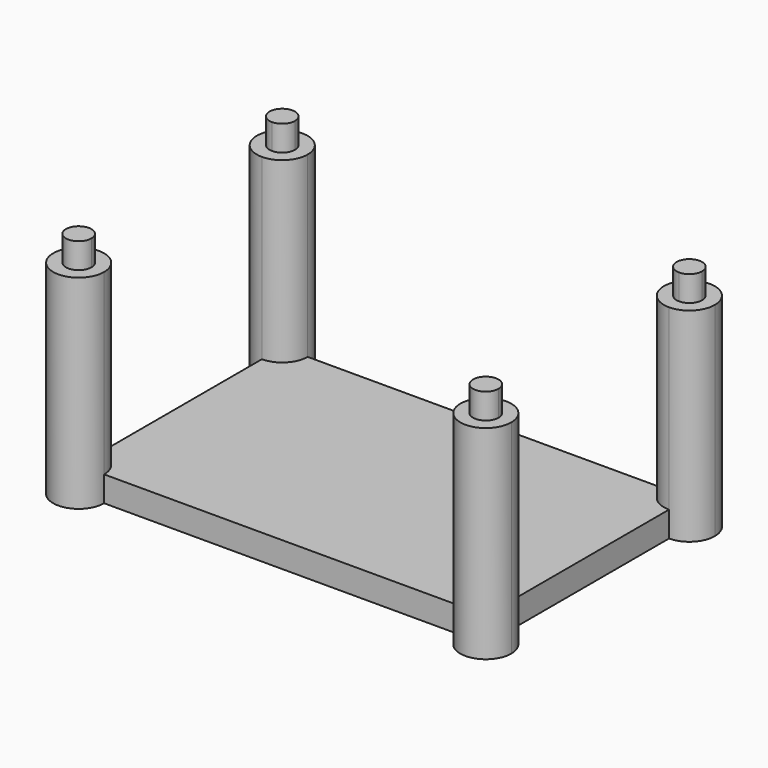
from build123d import *

# Parameters (mm, degrees)
F1_DEPTH   = 50.8
F2_DEPTH   = 6.35
F3_DEPTH   = 57.15
F4_D       = 7.62
F4_DEPTH   = 7.62
F4_TIP     = 2.2892789585
F4_2_D     = 7.62
F4_2_DEPTH = 7.62
F4_2_TIP   = 2.2892789585
F4_3_D     = 7.62
F4_3_DEPTH = 7.62
F4_3_TIP   = 2.2892789585
F4_4_D     = 7.62
F4_4_DEPTH = 7.62
F4_4_TIP   = 2.2892789585
F4_5_D     = 7.62
F4_5_DEPTH = 7.62
F4_5_TIP   = 2.2892789585
F4_6_D     = 7.62
F4_6_DEPTH = 7.62
F4_6_TIP   = 2.2892789585
F4_7_D     = 7.62
F4_7_DEPTH = 7.62
F4_7_TIP   = 2.2892789585
F4_8_D     = 7.62
F4_8_DEPTH = 7.62
F4_8_TIP   = 2.2892789585


with BuildPart() as f1:
    # F0 (on Top) → F1 (new body)
    with BuildSketch(Plane.XY):
        with BuildLine():
            Line((-47.625, 31.75), (-44.45, 31.75))
            ThreePointArc((-44.45, 31.75), (-55.2901280605, 36.2401280605), (-50.8, 25.4))
            Line((-50.8, 25.4), (-50.8, 28.575))
            ThreePointArc((-50.8, 28.575), (-53.0450640303, 33.9950640303), (-47.625, 31.75))
        make_face()
        with BuildLine():
            Line((-50.8, 31.75), (-47.625, 31.75))
            ThreePointArc((-47.625, 31.75), (-53.0450640303, 33.9950640303), (-50.8, 28.575))
            Line((-50.8, 28.575), (-50.8, 31.75))
        make_face()
        with BuildLine():
            ThreePointArc((-50.8, 28.575), (-48.5549359697, 29.5049359697), (-47.625, 31.75))
            Line((-47.625, 31.75), (-50.8, 31.75))
            Line((-50.8, 31.75), (-50.8, 28.575))
        make_face()
        with BuildLine():
            ThreePointArc((-50.8, 25.4), (-46.3098719395, 27.2598719395), (-44.45, 31.75))
            Line((-44.45, 31.75), (-47.625, 31.75))
            ThreePointArc((-47.625, 31.75), (-48.5549359697, 29.5049359697), (-50.8, 28.575))
            Line((-50.8, 28.575), (-50.8, 25.4))
        make_face()
    extrude(amount=F1_DEPTH)

    # F4
    with Locations(Plane(origin=(0, 0, 0), x_dir=(1, 0, 0), z_dir=(0, 0, -1))):
        with Locations((-50.8, 31.75), (-50.8, -31.75), (50.8, -31.75), (50.8, 31.75)):
            Hole(F4_D / 2, depth=F4_DEPTH)
            with Locations((0, 0, -(F4_DEPTH + F4_TIP / 2))):  # 118° drill point
                Cone(0, F4_D / 2, F4_TIP, mode=Mode.SUBTRACT)


with BuildPart() as f1b:
    # F0 (on Top) → F1, piece 2 (new body)
    with BuildSketch(Plane.XY):
        with BuildLine():
            Line((47.625, 31.75), (44.45, 31.75))
            ThreePointArc((44.45, 31.75), (46.3098719395, 27.2598719395), (50.8, 25.4))
            Line((50.8, 25.4), (50.8, 28.575))
            ThreePointArc((50.8, 28.575), (48.5549359697, 29.5049359697), (47.625, 31.75))
        make_face()
        with BuildLine():
            Line((50.8, 31.75), (47.625, 31.75))
            ThreePointArc((47.625, 31.75), (48.5549359697, 29.5049359697), (50.8, 28.575))
            Line((50.8, 28.575), (50.8, 31.75))
        make_face()
        with BuildLine():
            ThreePointArc((57.15, 31.75), (50.8, 38.1), (44.45, 31.75))
            Line((44.45, 31.75), (47.625, 31.75))
            ThreePointArc((47.625, 31.75), (50.8, 34.925), (53.975, 31.75))
            ThreePointArc((53.975, 31.75), (53.0450640303, 29.5049359697), (50.8, 28.575))
            Line((50.8, 28.575), (50.8, 25.4))
            ThreePointArc((50.8, 25.4), (55.2901280605, 27.2598719395), (57.15, 31.75))
        make_face()
        with BuildLine():
            ThreePointArc((53.975, 31.75), (50.8, 34.925), (47.625, 31.75))
            Line((47.625, 31.75), (50.8, 31.75))
            Line((50.8, 31.75), (50.8, 28.575))
            ThreePointArc((50.8, 28.575), (53.0450640303, 29.5049359697), (53.975, 31.75))
        make_face()
    extrude(amount=F1_DEPTH)

    # F4#2
    with Locations(Plane(origin=(0, 0, 0), x_dir=(1, 0, 0), z_dir=(0, 0, -1))):
        with Locations((-50.8, 31.75), (-50.8, -31.75), (50.8, -31.75), (50.8, 31.75)):
            Hole(F4_2_D / 2, depth=F4_2_DEPTH)
            with Locations((0, 0, -(F4_2_DEPTH + F4_2_TIP / 2))):  # 118° drill point
                Cone(0, F4_2_D / 2, F4_2_TIP, mode=Mode.SUBTRACT)


with BuildPart() as f1c:
    # F0 (on Top) → F1, piece 3 (new body)
    with BuildSketch(Plane.XY):
        with BuildLine():
            Line((50.8, -28.575), (50.8, -25.4))
            ThreePointArc((50.8, -25.4), (46.3098719395, -27.2598719395), (44.45, -31.75))
            Line((44.45, -31.75), (47.625, -31.75))
            ThreePointArc((47.625, -31.75), (48.5549359697, -29.5049359697), (50.8, -28.575))
        make_face()
        with BuildLine():
            ThreePointArc((57.15, -31.75), (55.2901280605, -27.2598719395), (50.8, -25.4))
            Line((50.8, -25.4), (50.8, -28.575))
            ThreePointArc((50.8, -28.575), (53.0450640303, -29.5049359697), (53.975, -31.75))
            ThreePointArc((53.975, -31.75), (50.8, -34.925), (47.625, -31.75))
            Line((47.625, -31.75), (44.45, -31.75))
            ThreePointArc((44.45, -31.75), (50.8, -38.1), (57.15, -31.75))
        make_face()
        with BuildLine():
            ThreePointArc((53.975, -31.75), (53.0450640303, -29.5049359697), (50.8, -28.575))
            Line((50.8, -28.575), (50.8, -31.75))
            Line((50.8, -31.75), (47.625, -31.75))
            ThreePointArc((47.625, -31.75), (50.8, -34.925), (53.975, -31.75))
        make_face()
        with BuildLine():
            Line((50.8, -31.75), (50.8, -28.575))
            ThreePointArc((50.8, -28.575), (48.5549359697, -29.5049359697), (47.625, -31.75))
            Line((47.625, -31.75), (50.8, -31.75))
        make_face()
    extrude(amount=F1_DEPTH)

    # F4#3
    with Locations(Plane(origin=(0, 0, 0), x_dir=(1, 0, 0), z_dir=(0, 0, -1))):
        with Locations((-50.8, 31.75), (-50.8, -31.75), (50.8, -31.75), (50.8, 31.75)):
            Hole(F4_3_D / 2, depth=F4_3_DEPTH)
            with Locations((0, 0, -(F4_3_DEPTH + F4_3_TIP / 2))):  # 118° drill point
                Cone(0, F4_3_D / 2, F4_3_TIP, mode=Mode.SUBTRACT)


with BuildPart() as f1d:
    # F0 (on Top) → F1, piece 4 (new body)
    with BuildSketch(Plane.XY):
        with BuildLine():
            Line((-50.8, -28.575), (-50.8, -25.4))
            ThreePointArc((-50.8, -25.4), (-55.2901280605, -36.2401280605), (-44.45, -31.75))
            Line((-44.45, -31.75), (-47.625, -31.75))
            ThreePointArc((-47.625, -31.75), (-53.0450640303, -33.9950640303), (-50.8, -28.575))
        make_face()
        with BuildLine():
            Line((-50.8, -31.75), (-50.8, -28.575))
            ThreePointArc((-50.8, -28.575), (-53.0450640303, -33.9950640303), (-47.625, -31.75))
            Line((-47.625, -31.75), (-50.8, -31.75))
        make_face()
        with BuildLine():
            ThreePointArc((-47.625, -31.75), (-48.5549359697, -29.5049359697), (-50.8, -28.575))
            Line((-50.8, -28.575), (-50.8, -31.75))
            Line((-50.8, -31.75), (-47.625, -31.75))
        make_face()
        with BuildLine():
            ThreePointArc((-44.45, -31.75), (-46.3098719395, -27.2598719395), (-50.8, -25.4))
            Line((-50.8, -25.4), (-50.8, -28.575))
            ThreePointArc((-50.8, -28.575), (-48.5549359697, -29.5049359697), (-47.625, -31.75))
            Line((-47.625, -31.75), (-44.45, -31.75))
        make_face()
    extrude(amount=F1_DEPTH)

    # F4#4
    with Locations(Plane(origin=(0, 0, 0), x_dir=(1, 0, 0), z_dir=(0, 0, -1))):
        with Locations((-50.8, 31.75), (-50.8, -31.75), (50.8, -31.75), (50.8, 31.75)):
            Hole(F4_4_D / 2, depth=F4_4_DEPTH)
            with Locations((0, 0, -(F4_4_DEPTH + F4_4_TIP / 2))):  # 118° drill point
                Cone(0, F4_4_D / 2, F4_4_TIP, mode=Mode.SUBTRACT)


with BuildPart() as f2:
    # F0 (on Top) → F2 (new body)
    with BuildSketch(Plane.XY):
        with BuildLine():
            Line((44.45, 31.75), (-44.45, 31.75))
            ThreePointArc((-44.45, 31.75), (-46.3098719395, 27.2598719395), (-50.8, 25.4))
            Line((-50.8, 25.4), (-50.8, -25.4))
            ThreePointArc((-50.8, -25.4), (-46.3098719395, -27.2598719395), (-44.45, -31.75))
            Line((-44.45, -31.75), (44.45, -31.75))
            ThreePointArc((44.45, -31.75), (46.3098719395, -27.2598719395), (50.8, -25.4))
            Line((50.8, -25.4), (50.8, 25.4))
            ThreePointArc((50.8, 25.4), (46.3098719395, 27.2598719395), (44.45, 31.75))
        make_face()
    extrude(amount=F2_DEPTH)


with BuildPart() as f3:
    # F0 (on Top) → F3 (new body)
    with BuildSketch(Plane.XY):
        with BuildLine():
            Line((-50.8, -31.75), (-50.8, -28.575))
            ThreePointArc((-50.8, -28.575), (-53.0450640303, -33.9950640303), (-47.625, -31.75))
            Line((-47.625, -31.75), (-50.8, -31.75))
        make_face()
        with BuildLine():
            ThreePointArc((-47.625, -31.75), (-48.5549359697, -29.5049359697), (-50.8, -28.575))
            Line((-50.8, -28.575), (-50.8, -31.75))
            Line((-50.8, -31.75), (-47.625, -31.75))
        make_face()
    extrude(amount=F3_DEPTH)

    # F4#5
    with Locations(Plane(origin=(0, 0, 0), x_dir=(1, 0, 0), z_dir=(0, 0, -1))):
        with Locations((-50.8, 31.75), (-50.8, -31.75), (50.8, -31.75), (50.8, 31.75)):
            Hole(F4_5_D / 2, depth=F4_5_DEPTH)
            with Locations((0, 0, -(F4_5_DEPTH + F4_5_TIP / 2))):  # 118° drill point
                Cone(0, F4_5_D / 2, F4_5_TIP, mode=Mode.SUBTRACT)


with BuildPart() as f3b:
    # F0 (on Top) → F3, piece 2 (new body)
    with BuildSketch(Plane.XY):
        with BuildLine():
            Line((-50.8, 31.75), (-47.625, 31.75))
            ThreePointArc((-47.625, 31.75), (-53.0450640303, 33.9950640303), (-50.8, 28.575))
            Line((-50.8, 28.575), (-50.8, 31.75))
        make_face()
        with BuildLine():
            ThreePointArc((-50.8, 28.575), (-48.5549359697, 29.5049359697), (-47.625, 31.75))
            Line((-47.625, 31.75), (-50.8, 31.75))
            Line((-50.8, 31.75), (-50.8, 28.575))
        make_face()
    extrude(amount=F3_DEPTH)

    # F4#6
    with Locations(Plane(origin=(0, 0, 0), x_dir=(1, 0, 0), z_dir=(0, 0, -1))):
        with Locations((-50.8, 31.75), (-50.8, -31.75), (50.8, -31.75), (50.8, 31.75)):
            Hole(F4_6_D / 2, depth=F4_6_DEPTH)
            with Locations((0, 0, -(F4_6_DEPTH + F4_6_TIP / 2))):  # 118° drill point
                Cone(0, F4_6_D / 2, F4_6_TIP, mode=Mode.SUBTRACT)


with BuildPart() as f3c:
    # F0 (on Top) → F3, piece 3 (new body)
    with BuildSketch(Plane.XY):
        with BuildLine():
            ThreePointArc((53.975, 31.75), (50.8, 34.925), (47.625, 31.75))
            Line((47.625, 31.75), (50.8, 31.75))
            Line((50.8, 31.75), (50.8, 28.575))
            ThreePointArc((50.8, 28.575), (53.0450640303, 29.5049359697), (53.975, 31.75))
        make_face()
        with BuildLine():
            Line((50.8, 31.75), (47.625, 31.75))
            ThreePointArc((47.625, 31.75), (48.5549359697, 29.5049359697), (50.8, 28.575))
            Line((50.8, 28.575), (50.8, 31.75))
        make_face()
    extrude(amount=F3_DEPTH)

    # F4#7
    with Locations(Plane(origin=(0, 0, 0), x_dir=(1, 0, 0), z_dir=(0, 0, -1))):
        with Locations((-50.8, 31.75), (-50.8, -31.75), (50.8, -31.75), (50.8, 31.75)):
            Hole(F4_7_D / 2, depth=F4_7_DEPTH)
            with Locations((0, 0, -(F4_7_DEPTH + F4_7_TIP / 2))):  # 118° drill point
                Cone(0, F4_7_D / 2, F4_7_TIP, mode=Mode.SUBTRACT)


with BuildPart() as f3d:
    # F0 (on Top) → F3, piece 4 (new body)
    with BuildSketch(Plane.XY):
        with BuildLine():
            ThreePointArc((53.975, -31.75), (53.0450640303, -29.5049359697), (50.8, -28.575))
            Line((50.8, -28.575), (50.8, -31.75))
            Line((50.8, -31.75), (47.625, -31.75))
            ThreePointArc((47.625, -31.75), (50.8, -34.925), (53.975, -31.75))
        make_face()
        with BuildLine():
            Line((50.8, -31.75), (50.8, -28.575))
            ThreePointArc((50.8, -28.575), (48.5549359697, -29.5049359697), (47.625, -31.75))
            Line((47.625, -31.75), (50.8, -31.75))
        make_face()
    extrude(amount=F3_DEPTH)

    # F4#8
    with Locations(Plane(origin=(0, 0, 0), x_dir=(1, 0, 0), z_dir=(0, 0, -1))):
        with Locations((-50.8, 31.75), (-50.8, -31.75), (50.8, -31.75), (50.8, 31.75)):
            Hole(F4_8_D / 2, depth=F4_8_DEPTH)
            with Locations((0, 0, -(F4_8_DEPTH + F4_8_TIP / 2))):  # 118° drill point
                Cone(0, F4_8_D / 2, F4_8_TIP, mode=Mode.SUBTRACT)


solid = Compound([f1.part, f1b.part, f1c.part, f1d.part, f2.part, f3.part, f3b.part, f3c.part, f3d.part])
